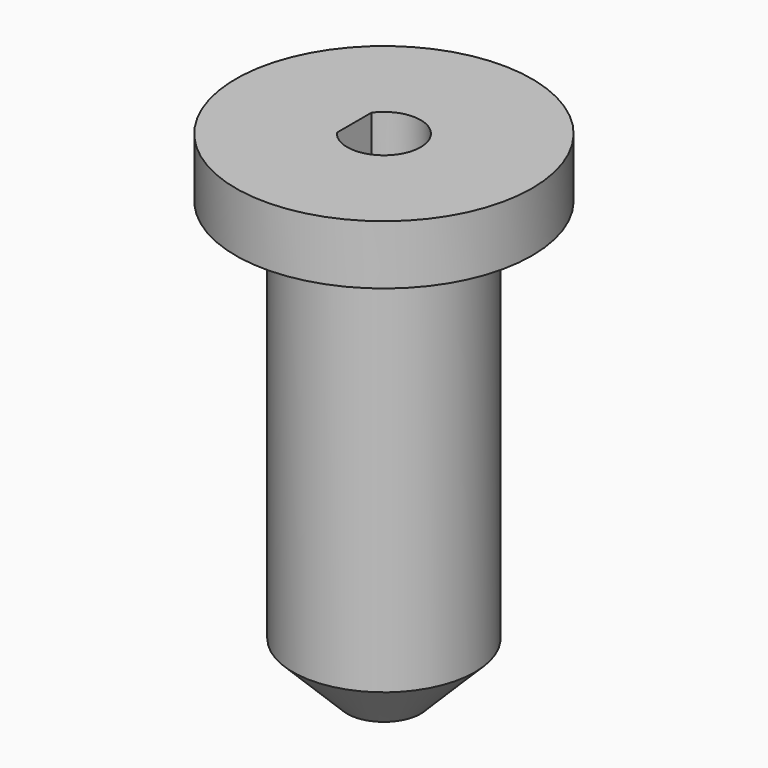
from build123d import *

# Parameters (mm, degrees)
F1_R     = 7.8105
F2_DEPTH = 38.1
F3_DEPTH = 50.8
F4_R     = 12.7
F4_R_2   = 7.8105
F5_DEPTH = 5.08


# Not quite as in the source:
# - a fillet or chamfer that OpenCascade refuses, or shapes differently, is made with other operations: its cross-section is extruded or revolved along the edge and cut away or added


with BuildPart() as f2:
    # F1 (on Top) → F2 (new body)
    with BuildSketch(Plane.XY):
        Circle(F1_R)
    extrude(amount=F2_DEPTH)

    # F0 (on Top) → F3 (cut)
    with BuildSketch(Plane.XY):
        with BuildLine():
            Line((-2.55, 1.8493242009), (-2.55, -1.8493242009))
            ThreePointArc((-2.55, -1.8493242009), (3.15, 0), (-2.55, 1.8493242009))
        make_face()
    extrude(amount=F3_DEPTH, mode=Mode.SUBTRACT)

    # F4 (on face) → F5 (join)
    with BuildSketch(Plane.XY.offset(38.1)):
        Circle(F4_R)
        Circle(F4_R_2, mode=Mode.SUBTRACT)
        Circle(F4_R_2)
        with BuildLine():
            Line((-2.55, -1.8493242009), (-2.55, 1.8493242009))
            ThreePointArc((-2.55, 1.8493242009), (3.15, 0), (-2.55, -1.8493242009))
        make_face(mode=Mode.SUBTRACT)
    extrude(amount=F5_DEPTH)

    # F6: chamfer of 5.08 on 1 edges, made by hand

    # F6_s1 → F6_t2 (revolve, cut)
    with BuildSketch(Plane.XZ):
        Polygon((7.8105, 5.08), (2.7305, 0), (7.8105, 0), align=None)
    revolve(axis=Axis((0, 0, 0), (0, 0, 1)), mode=Mode.SUBTRACT)


solid = f2.part
